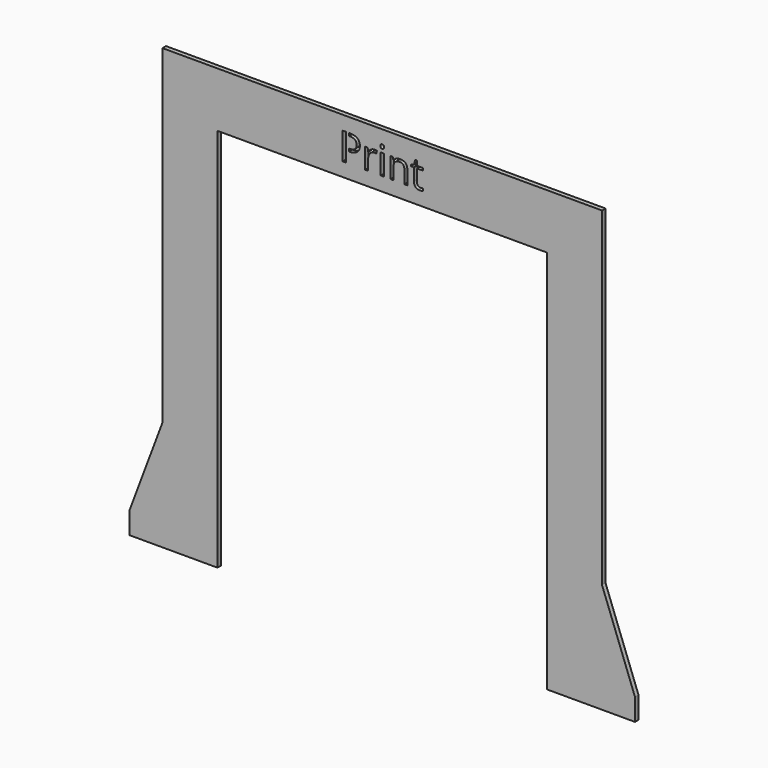
from build123d import *

# Parameters (mm, degrees)
F1_DEPTH     = 4
F2_TEXT_SIZE = 34.7222222222
F3_DEPTH     = 25
F4_W         = 3
F4_H         = 15.0390625
F5_DEPTH     = 4


# Not quite as in the source:
# - Text() gives the source's letters only with a copy of the font that has no kerning and outlines rounded to 1/6400 em; it was checked with that copy


with BuildPart() as f1:
    # F0 (on Front) → F1 (new body)
    with BuildSketch(Plane.XZ):
        Polygon((-150, -350), (-150, 0), (150, 0), (150, -350), (230, -350), (230, -330), (200, -250), (200, 50), (-200, 50), (-200, -250), (-230, -330), (-230, -350), align=None)
    extrude(amount=F1_DEPTH)

    # F2 (on face) → F3 (cut)
    with BuildSketch(Plane.XZ.offset(4)):
        with Locations((-39.4775390625, 12.5)):
            Text('Print', F2_TEXT_SIZE, font='Open Sans', text_align=(TextAlign.LEFT, TextAlign.BOTTOM))
    extrude(amount=-F3_DEPTH, mode=Mode.SUBTRACT)

    # F4 (on face) → F5 (join)
    with BuildSketch(Plane.XZ.offset(4)):
        with Locations((-31.6895616319, 29.7688802083)):
            Rectangle(F4_W, F4_H)
    extrude(amount=-F5_DEPTH)


solid = f1.part
